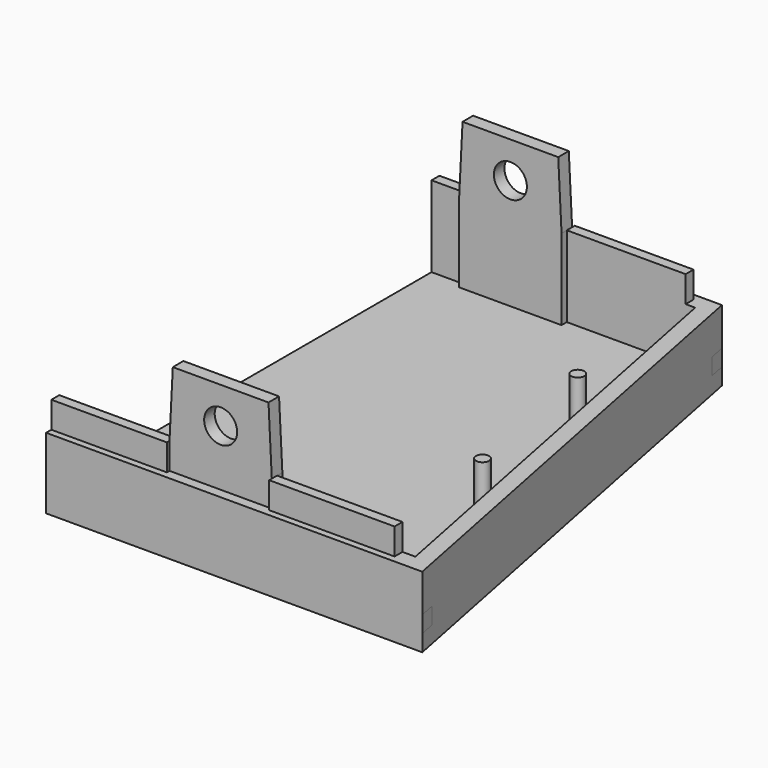
from build123d import *

# Parameters (mm, degrees)
F0_W           = 42
F0_H           = 75.5
F1_DEPTH       = 2.5
F3_DEPTH       = 2.5
F5_DEPTH       = 5.75
F8_DEPTH       = 1
F9_W           = 38.5
F9_H           = 1.5
F9_W_2         = 52
F10_DEPTH      = 4
F11_W          = 15.5
F11_H          = 4
F12_DEPTH      = 0.5
F13_W          = 15.5
F13_H          = 4
F14_DEPTH      = 0.5
F15_W          = 15.5
F15_H          = 1
F15_H_2        = 2
F16_DEPTH      = 14.5
F16_DEPTH_BACK = 10
F17_SIZE2      = 0.49999
F17_SIZE       = 9.99999
F17_2_SIZE2    = 0.49999
F17_2_SIZE     = 9.99999
F18_SIZE2      = 9.99999
F18_SIZE       = 0.49999
F19_R          = 2.5
F20_DEPTH      = 2
F21_R          = 2.5
F22_DEPTH      = 2
F23_R          = 1
F24_DEPTH      = 10


# Not quite as in the source:
# - a fillet or chamfer is up to 0.001 mm smaller than in the source, because OpenCascade refuses the exact size
# - a feature names something its author has since deleted; it is built from what else it names


with BuildPart() as f1:
    # F0 (on Top) → F1 (new body)
    with BuildSketch(Plane.XY):
        Rectangle(F0_W, F0_H)
        Polygon((21, 37.75), (21, -37.75), (36, -37.75), align=None)
    extrude(amount=F1_DEPTH)

    # F2 (on face) → F3 (join)
    with BuildSketch(Plane.XY.offset(2.5)):
        Polygon((21.4966887417, 35.25), (18.947826308, 35.25), (32.9544488245, -35.25), (35.5033112583, -35.25), align=None)
        Polygon((18.4511375663, 37.75), (-21, 37.75), (-21, 35.25), (18.947826308, 35.25), align=None)
        Polygon((32.9544488245, -35.25), (-21, -35.25), (-21, -37.75), (33.4511375663, -37.75), align=None)
        Polygon((21, 37.75), (18.4511375663, 37.75), (18.947826308, 35.25), (21.4966887417, 35.25), align=None)
        Polygon((35.5033112583, -35.25), (32.9544488245, -35.25), (33.4511375663, -37.75), (36, -37.75), align=None)
    extrude(amount=F3_DEPTH)

    # F4 (on face) → F5 (join)
    with BuildSketch(Plane.XY.offset(5)):
        Polygon((-21, 35.25), (18.947826308, 35.25), (32.9544488245, -35.25), (-21, -35.25), (-21, -37.75), (36, -37.75), (21, 37.75), (-21, 37.75), align=None)
    extrude(amount=F5_DEPTH)

    # F7 (on face) → F8 (cut)
    with BuildSketch(Plane(origin=(0, 37.75, 0), x_dir=(-1, 0, 0), z_dir=(0, 1, 0))):
        Polygon((21, 5), (21, 10.75), (17, 10.75), (17.25, 5), align=None)
    extrude(amount=-F8_DEPTH, mode=Mode.SUBTRACT)

    # F9 (on face) → F10 (join)
    with BuildSketch(Plane.XY.offset(10.75)):
        with Locations((-1.75, 36)):
            Rectangle(F9_W, F9_H)
        with Locations((5, -36)):
            Rectangle(F9_W_2, F9_H)
    extrude(amount=F10_DEPTH)

    # F11 (on face) → F12 (cut)
    with BuildSketch(Plane.XZ.offset(36.75)):
        with Locations((4.25, 12.75)):
            Rectangle(F11_W, F11_H)
    extrude(amount=-F12_DEPTH, mode=Mode.SUBTRACT)

    # F13 (on face) → F14 (cut)
    with BuildSketch(Plane(origin=(0, 36.75, 0), x_dir=(-1, 0, 0), z_dir=(0, 1, 0))):
        with Locations((8.25, 12.75)):
            Rectangle(F13_W, F13_H)
    extrude(amount=-F14_DEPTH, mode=Mode.SUBTRACT)

    # F15 (on face) → F16 (join, two sides)
    with BuildSketch(Plane.XY.offset(14.75)) as f16_sk:
        with Locations((4.25, -35.75)):
            Rectangle(F15_W, F15_H)
        with Locations((4.25, -34.75)):
            Rectangle(F15_W, F15_H)
        with Locations((-8.25, 35.25)):
            Rectangle(F15_W, F15_H_2)
    extrude(amount=-F16_DEPTH)
    extrude(f16_sk.sketch, amount=F16_DEPTH_BACK)

    # F17 (size 10 and 0.5 in the source; OpenCascade refuses exactly that, so slightly less here)
    f17_edges = [f1.edges().sort_by_distance(p)[0] for p in [
        (-0.5, 35.25, 24.75),
    ]]
    f17_side = f1.faces().sort_by_distance((-0.5, 35.060078, 15.524225))[0]
    chamfer(f17_edges, length=F17_SIZE, length2=F17_SIZE2, reference=f17_side)

    # F17#2 (size 10 and 0.5 in the source; OpenCascade refuses exactly that, so slightly less here)
    f17_2_edges = [f1.edges().sort_by_distance(p)[0] for p in [
        (-16, 35.25, 24.75),
    ]]
    f17_2_side = f1.faces().sort_by_distance((-16, 35.060078, 15.524225))[0]
    chamfer(f17_2_edges, length=F17_2_SIZE, length2=F17_2_SIZE2, reference=f17_2_side)

    # F18 (size 0.5 and 10 in the source; OpenCascade refuses exactly that, so slightly less here)
    f18_edges = [f1.edges().sort_by_distance(p)[0] for p in [
        (12, -35.25, 24.75),
        (-3.5, -35.25, 24.75),
    ]]
    f18_side = f1.faces().sort_by_distance((4.25, -35.25, 24.75))[0]
    chamfer(f18_edges, length=F18_SIZE, length2=F18_SIZE2, reference=f18_side)

    # F19 (on face) → F20 (cut, through all)
    with BuildSketch(Plane(origin=(0, 36.25, 0), x_dir=(-1, 0, 0), z_dir=(0, 1, 0))):
        with Locations((8.25, 19.25)):
            Circle(F19_R)
    extrude(amount=-F20_DEPTH, mode=Mode.SUBTRACT)

    # F21 (on face) → F22 (cut, through all)
    with BuildSketch(Plane.XZ.offset(36.25)):
        with Locations((4.25, 19.25)):
            Circle(F21_R)
    extrude(amount=-F22_DEPTH, mode=Mode.SUBTRACT)

    # F23 (on face) → F24 (join)
    with BuildSketch(Plane.XY.offset(2.5)):
        with Locations((20.7567410564, 10.75)):
            Circle(F23_R)
        with Locations((25.5249529769, -13.25)):
            Circle(F23_R)
    extrude(amount=F24_DEPTH)


solid = f1.part
